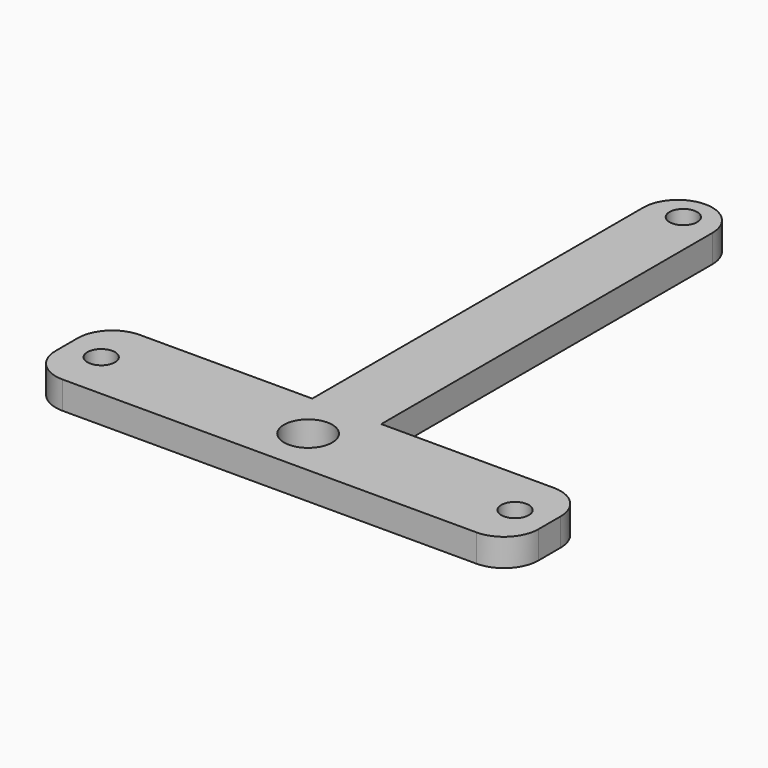
from build123d import *

# Parameters (mm, degrees)
F1_DEPTH = 4
F2_R     = 2
F2_R_2   = 3.5
F3_DEPTH = 25
F4_R     = 4.99999


# Not quite as in the source:
# - a fillet or chamfer is up to 0.001 mm smaller than in the source, because OpenCascade refuses the exact size


with BuildPart() as f1:
    # F0 (on Top) → F1 (new body)
    with BuildSketch(Plane.XY):
        Polygon((-5, 65), (-5, 0), (-35, 0), (-35, -14), (35, -14), (35, 0), (5, 0), (5, 65), align=None)
    extrude(amount=F1_DEPTH)

    # F2 (on face) → F3 (cut)
    with BuildSketch(Plane.XY.offset(4)):
        with Locations((-30, -7)):
            Circle(F2_R)
        with Locations((30, -7)):
            Circle(F2_R)
        with Locations((0, -7)):
            Circle(F2_R_2)
        with Locations((0, 61)):
            Circle(F2_R)
    extrude(amount=-F3_DEPTH, mode=Mode.SUBTRACT)

    # F4 (radius 5 in the source; OpenCascade refuses exactly that, so slightly less here)
    f4_edges = [f1.edges().sort_by_distance(p)[0] for p in [
        (-35, -14, 2),
        (-35, 0, 2),
        (35, -14, 2),
        (35, 0, 2),
        (5, 65, 2),
        (-5, 65, 2),
    ]]
    fillet(f4_edges, radius=F4_R)


solid = f1.part
